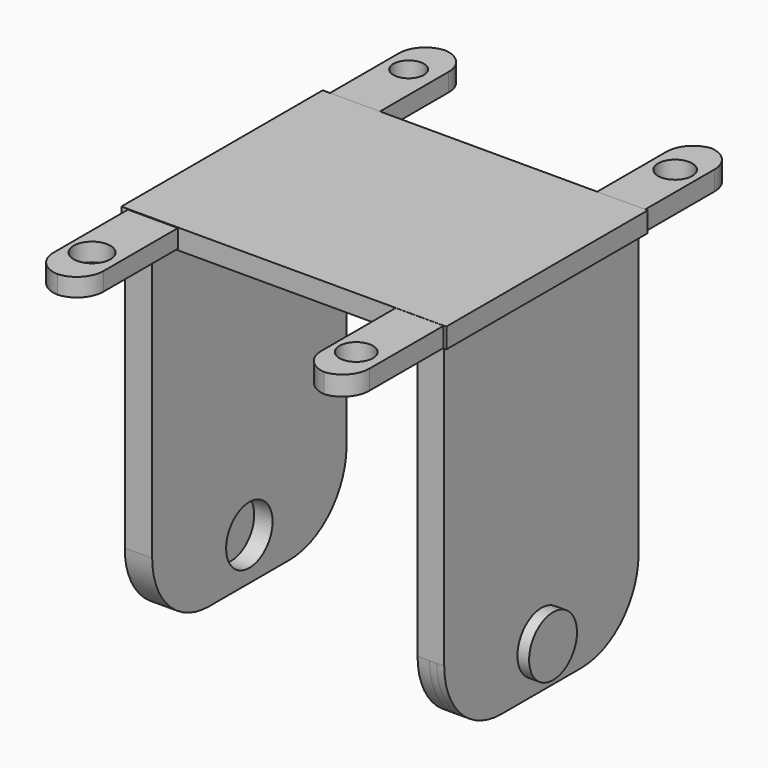
from build123d import *

# Parameters (mm, degrees)
F0_W         = 77.900249511
F0_H         = 6.2239915133
F1_DEPTH     = 50.292
F2_W         = 5.9690438211
F2_H         = 109.3528494239
F2_W_2       = 6.2078051269
F2_H_2       = 109.8303757608
F3_DEPTH     = 37.592
F4_R         = 22.0755688143
F5_DEPTH     = 2.286
F7_R         = 9.5028337992
F8_DEPTH     = 3.6
F6_R         = 9.2619968466
F9_DEPTH     = 3.6
F10_R        = 8.2457773543
F12_DEPTH    = 7.7
F11_R        = 8.9872233932
F13_DEPTH    = 5.7
F14_W        = 14.8572660983
F14_H        = 6.0232169926
F14_W_2      = 15.4595859349
F14_H_2      = 5.6216679513
F15_DEPTH    = 75
F16_T1_DEPTH = 46.6632985117
F16_T3_DEPTH = 47.064847553
F17_R        = 4.7067592452
F17_R_2      = 5.2876360091
F17_R_3      = 5.6910023403
F17_R_4      = 5.1821036644
F18_DEPTH    = 25


# Not quite as in the source:
# - a fillet or chamfer that OpenCascade refuses, or shapes differently, is made with other operations: its cross-section is extruded or revolved along the edge and cut away or added


with BuildPart() as f1:
    # F0 (on Right) → F1 (new body, symmetric)
    with BuildSketch(Plane.YZ):
        with Locations((0.9574238211, 36.620259285)):
            Rectangle(F0_W, F0_H)
    extrude(amount=F1_DEPTH, both=True)

    # F2 (on Front) → F3 (join, symmetric)
    with BuildSketch(Plane.XZ):
        with Locations((44.0515298396, -20.6528864801)):
            Rectangle(F2_W, F2_H)
        with Locations((-44.1709104925, -20.4141233116)):
            Rectangle(F2_W_2, F2_H_2)
    extrude(amount=F3_DEPTH, both=True)

    # F4
    f4_edges = [f1.edges().sort_by_distance(p)[0] for p in [
        (44.05153, 37.592, -75.329311),
        (44.05153, -37.592, -75.329311),
        (-44.17091, -37.592, -75.329311),
        (-44.17091, 37.592, -75.329311),
    ]]
    fillet(f4_edges, radius=F4_R)

    # F5 (add, symmetric): faces of the model
    f5_faces = [f1.faces().sort_by_distance(p)[0] for p in [
        (47.0360517502, 0, -19.6123684117),
        (-47.274813056, 0, -19.6123684117),
    ]]
    extrude(f5_faces, amount=F5_DEPTH, both=True, dir=(1, 0, 0))

    # F7 (on face) → F8 (join)
    with BuildSketch(Plane(origin=(-49.560813056, 0, 0), x_dir=(0, -1, 0), z_dir=(-1, 0, 0))):
        with Locations((0, -61.9606114924)):
            Circle(F7_R)
    extrude(amount=F8_DEPTH)

    # F6 (on face) → F9 (join)
    with BuildSketch(Plane.YZ.offset(49.3220517502)):
        with Locations((0, -61.9290173054)):
            Circle(F6_R)
    extrude(amount=F9_DEPTH)

    # F10 (on face) → F12 (cut)
    with BuildSketch(Plane(origin=(41.0670079291, 0, 0), x_dir=(0, -1, 0), z_dir=(-1, 0, 0))):
        with Locations((0, -61.2058117986)):
            Circle(F10_R)
    extrude(amount=-F12_DEPTH, mode=Mode.SUBTRACT)

    # F11 (on face) → F13 (cut)
    with BuildSketch(Plane.YZ.offset(-41.0670079291)):
        with Locations((0, -62.1923357248)):
            Circle(F11_R)
    extrude(amount=-F13_DEPTH, mode=Mode.SUBTRACT)

    # F14 (on Front) → F15 (join, symmetric)
    with BuildSketch(Plane.XZ):
        with Locations((42.047848925, 36.6818103939)):
            Rectangle(F14_W, F14_H)
        with Locations((-40.5197497457, 36.7389488965)):
            Rectangle(F14_W_2, F14_H_2)
    extrude(amount=F15_DEPTH, both=True)

    # F16: fillet of radius 8.2083261121 on 8 edges, made by hand

    # F16_s2 → F16_t1 (cut)
    with BuildSketch(Plane.XY.offset(13.4072996407)):
        with BuildLine():
            ThreePointArc((-32.7899567783, 66.7916738879), (-35.1941198343, 72.595836944), (-40.9982828904, 75))
            Line((-40.9982828904, 75), (-32.7899567783, 75))
            Line((-32.7899567783, 75), (-32.7899567783, 66.7916738879))
        make_face()
        with BuildLine():
            ThreePointArc((-48.2495427132, 66.7916738879), (-45.8453796571, 72.595836944), (-40.0412166011, 75))
            Line((-40.0412166011, 75), (-48.2495427132, 75))
            Line((-48.2495427132, 75), (-48.2495427132, 66.7916738879))
        make_face()
        with BuildLine():
            ThreePointArc((-48.2495427132, -66.7916738879), (-45.8453796571, -72.595836944), (-40.0412166011, -75))
            Line((-40.0412166011, -75), (-48.2495427132, -75))
            Line((-48.2495427132, -75), (-48.2495427132, -66.7916738879))
        make_face()
        with BuildLine():
            ThreePointArc((-32.7899567783, -66.7916738879), (-35.1941198343, -72.595836944), (-40.9982828904, -75))
            Line((-40.9982828904, -75), (-32.7899567783, -75))
            Line((-32.7899567783, -75), (-32.7899567783, -66.7916738879))
        make_face()
    extrude(amount=F16_T1_DEPTH, mode=Mode.SUBTRACT)

    # F16_s4 → F16_t3 (cut)
    with BuildSketch(Plane.XY.offset(13.1493866174)):
        with BuildLine():
            ThreePointArc((49.4764819741, 66.7916738879), (47.0723189181, 72.595836944), (41.2681558621, 75))
            Line((41.2681558621, 75), (49.4764819741, 75))
            Line((49.4764819741, 75), (49.4764819741, 66.7916738879))
        make_face()
        with BuildLine():
            ThreePointArc((34.6192158759, 66.7916738879), (37.0233789319, 72.595836944), (42.8275419879, 75))
            Line((42.8275419879, 75), (34.6192158759, 75))
            Line((34.6192158759, 75), (34.6192158759, 66.7916738879))
        make_face()
        with BuildLine():
            ThreePointArc((49.4764819741, -66.7916738879), (47.0723189181, -72.595836944), (41.2681558621, -75))
            Line((41.2681558621, -75), (49.4764819741, -75))
            Line((49.4764819741, -75), (49.4764819741, -66.7916738879))
        make_face()
        with BuildLine():
            ThreePointArc((34.6192158759, -66.7916738879), (37.0233789319, -72.595836944), (42.8275419879, -75))
            Line((42.8275419879, -75), (34.6192158759, -75))
            Line((34.6192158759, -75), (34.6192158759, -66.7916738879))
        make_face()
    extrude(amount=F16_T3_DEPTH, mode=Mode.SUBTRACT)

    # F17 (on face) → F18 (cut)
    with BuildSketch(Plane.XY.offset(39.6934188902)):
        with Locations((-41.1323793232, 61.7104582489)):
            Circle(F17_R)
        with Locations((42.1323850751, 60.7389695942)):
            Circle(F17_R_2)
        with Locations((-41.0092622042, -60.9235055745)):
            Circle(F17_R_3)
        with Locations((41.5508002043, -61.9366765022)):
            Circle(F17_R_4)
    extrude(amount=-F18_DEPTH, mode=Mode.SUBTRACT)


solid = f1.part
